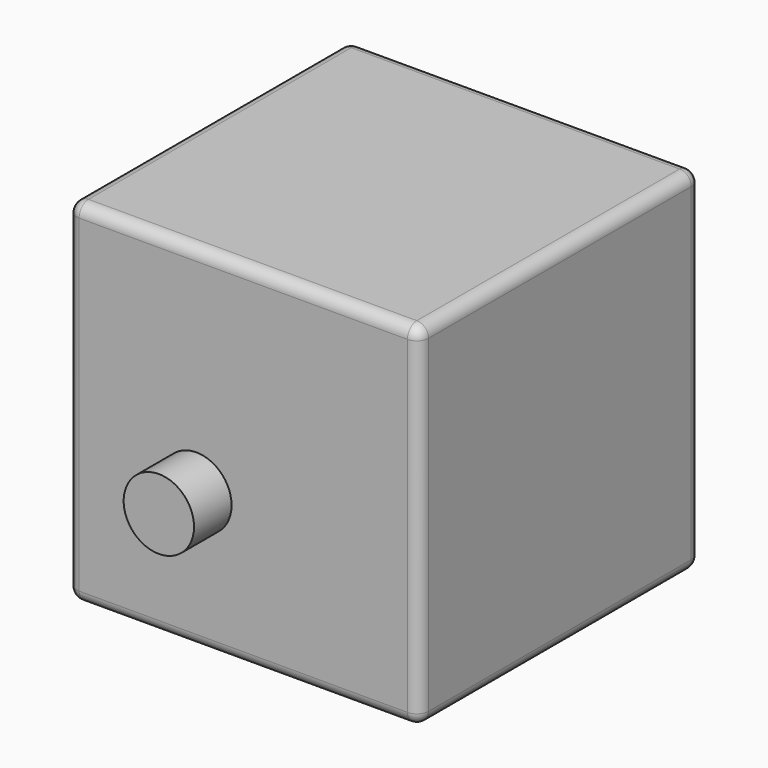
from build123d import *

# Parameters (mm, degrees)
F0_W      = 23.8125
F0_H      = 23.8125
F1_DEPTH  = 23.8125
F6_R      = 2.38125
F7_DEPTH  = 3.175
F9_R      = 3.96875
F10_DEPTH = 4.7625
F12_R     = 2.38125
F13_DEPTH = 3.175
F14_R     = 0.79375


# Not quite as in the source:
# - a length typed as a fraction of an inch, garbled in the dataset ("3 / 203.2 mm" for 3/8 in), is restored
# - the program builds the solid bodies; features that only make, move or delete a surface that nothing else refers to are left out


with BuildPart() as f1:
    # F0 (on Top) → F1 (new body)
    with BuildSketch(Plane.XY):
        with Locations((-2.8766207397, -2.0344056764)):
            Rectangle(F0_W, F0_H)
    extrude(amount=F1_DEPTH)

    # F9 (on offset) → F10 (join)
    with BuildSketch(Plane(origin=(0, 14.6343443236, 0), x_dir=(-1, 0, 0), z_dir=(0, 1, 0))):
        with Locations((2.8766207397, 11.90625)):
            Circle(F9_R)
    extrude(amount=-F10_DEPTH)

    # F12 (on offset) → F13 (join)
    with BuildSketch(Plane(origin=(0, 17.8093443236, 0), x_dir=(-1, 0, 0), z_dir=(0, 1, 0))):
        with Locations((2.8766207397, 11.90625)):
            Circle(F12_R)
    extrude(amount=-F13_DEPTH)

    # F14
    f14_edges = [f1.edges().sort_by_distance(p)[0] for p in [
        (9.029629, -2.034406, 0),
        (9.029629, -2.034406, 23.8125),
        (9.029629, -13.940656, 11.90625),
        (9.029629, 9.871844, 11.90625),
        (-2.876621, 9.871844, 23.8125),
        (-14.782871, -2.034406, 23.8125),
        (-2.876621, -13.940656, 23.8125),
        (-2.876621, 9.871844, 0),
        (-14.782871, 9.871844, 11.90625),
        (-14.782871, -13.940656, 11.90625),
        (-2.876621, -13.940656, 0),
        (-14.782871, -2.034406, 0),
    ]]
    fillet(f14_edges, radius=F14_R)


with BuildPart() as f7:
    # F6 (on offset) → F7 (new body)
    with BuildSketch(Plane.XZ.offset(21.0844056764)):
        with Locations((-2.8766207397, 11.90625)):
            Circle(F6_R)
    extrude(amount=-F7_DEPTH)


solid = Compound([f1.part, f7.part])
